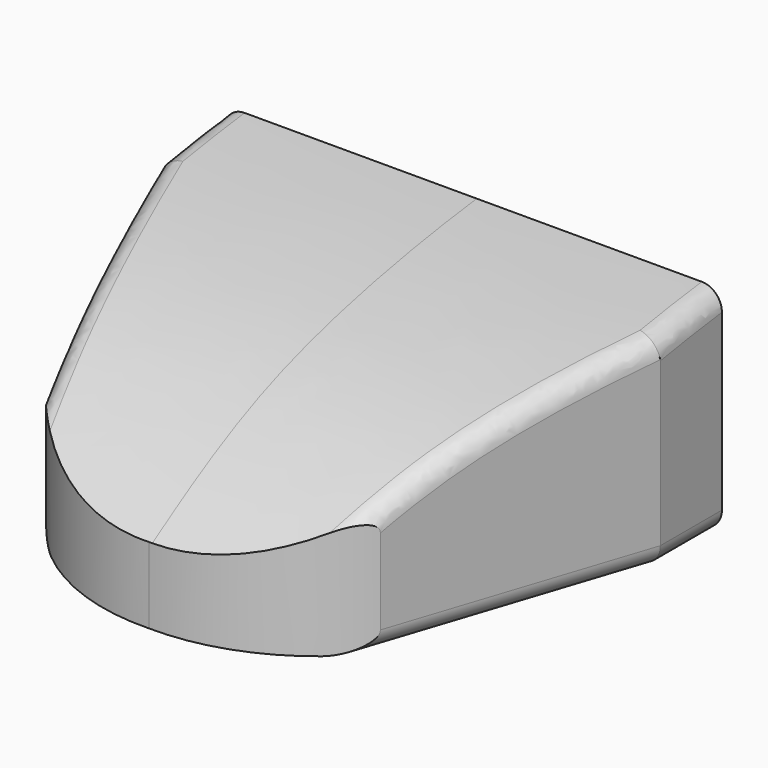
from build123d import *

# Parameters (mm, degrees)
F0_W     = 84.2862705333
F0_H     = 62.5252984464
F1_DEPTH = 38.1
F2_DEPTH = 19.431
F4_DEPTH = 76.2
F5_DEPTH = 50.8
F6_DEPTH = 19.05
F7_R     = 5.08


with BuildPart() as f1:
    # F0 (on Top) → F1 (new body)
    with BuildSketch(Plane.XY):
        with Locations((-0.8938079051, 9.4918403774)):
            Rectangle(F0_W, F0_H)
        Polygon((61.8553981185, 40.7544896007), (41.2493273616, 40.7544896007), (41.2493273616, -21.7708088458), align=None)
        Polygon((-43.0369431717, -21.7708088458), (-43.0369431717, 40.7544896007), (-63.6430233717, 40.7544896007), align=None)
        with BuildLine():
            Line((41.2493273616, -21.7708088458), (-43.0369431717, -21.7708088458))
            ThreePointArc((-43.0369431717, -21.7708088458), (-24.4435818385, -37.0758276989), (-0.8938079051, -42.1121791005))
            ThreePointArc((-0.8938079051, -42.1121791005), (22.5826118494, -36.9238529276), (41.2493273616, -21.7708088458))
        make_face()
    extrude(amount=F1_DEPTH)

    # F2 (add): a face of the model
    f2_faces = [f1.faces().sort_by_distance(p)[0] for p in [
        (-0.8938126266, 40.7544896007, 19.05),
    ]]
    extrude(f2_faces, amount=F2_DEPTH)

    # F3 (on Right) → F4 (join, symmetric)
    with BuildSketch(Plane.YZ):
        with BuildLine():
            add(Edge.make_bspline(
                [(-42.3909127712, 38.0631349981), (-29.9156566507, 46.1025365559), (-0.9292461645, 64.7821826505), (83.4228372852, 77.6600402112), (128.7347014113, 77.0774025905), (150.1817703247, 76.8016278744)],
                knots=[0, 0, 0, 0, 0.2846618796, 0.6614152802, 1, 1, 1, 1], degree=3))
            Line((-42.3909127712, 38.0631349981), (150.1817703247, 38.0631349981))
            Line((150.1817703247, 38.0631349981), (150.1817703247, 76.8016278744))
        make_face()
    extrude(amount=F4_DEPTH, both=True)

    # F5 (cut): a face of the model
    f5_faces = [f1.faces().sort_by_distance(p)[0] for p in [
        (0.4832953146, 74.166117784, 38.0631349981),
    ]]
    extrude(f5_faces, amount=-F5_DEPTH, mode=Mode.SUBTRACT)

    # F6 (cut): a face of the model
    f6_faces = [f1.faces().sort_by_distance(p)[0] for p in [
        (-0.9060877903, 15.8917005053, 0),
    ]]
    extrude(f6_faces, amount=-F6_DEPTH, mode=Mode.SUBTRACT)

    # F7
    f7_edges = [f1.edges().sort_by_distance(p)[0] for p in [
        (-53.339983, 9.49184, 19.05),
        (51.552363, 9.49184, 19.05),
        (51.296645, 8.715914, 63.106757),
        (0, 6.644686, 62.484239),
        (61.855398, 50.46999, 19.05),
        (-63.643023, 50.46999, 19.05),
        (61.855398, 50.453515, 71.874141),
        (-63.643023, 50.453515, 71.874141),
        (-53.105319, 8.779795, 63.12556),
    ]]
    fillet(f7_edges, radius=F7_R)


solid = f1.part
